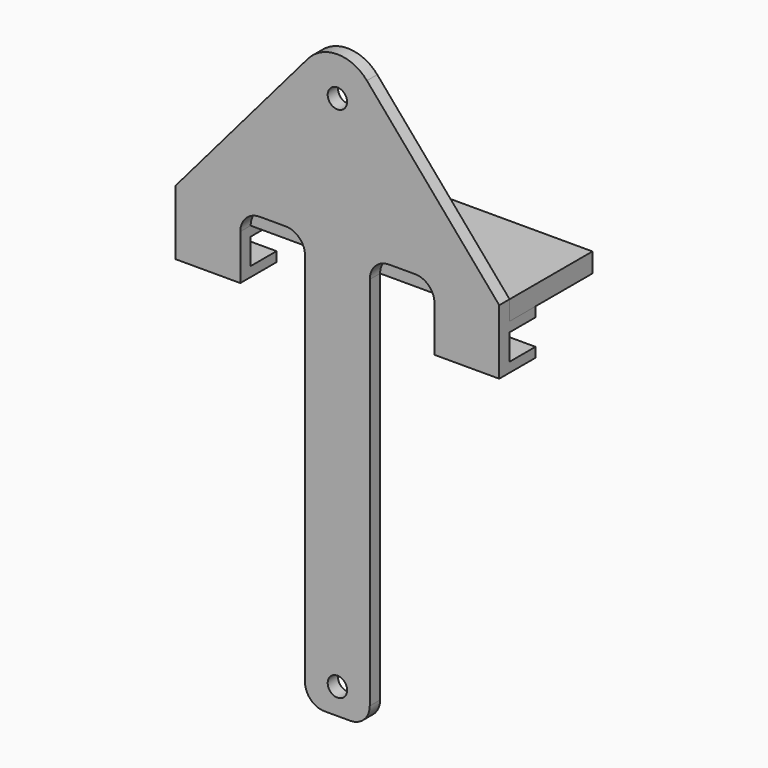
from build123d import *

# Parameters (mm, degrees)
F0_R     = 7.5
F1_DEPTH = 10
F2_W     = 50
F2_H     = 35
F3_DEPTH = 25
F5_DEPTH = 250.001
F6_W     = 250
F6_H     = 15
F7_DEPTH = 80


with BuildPart() as f1:
    # F0 (on Front) → F1 (new body)
    with BuildSketch(Plane.XZ):
        with BuildLine():
            Line((125, 50), (22.7990460802, 169.4988076003))
            ThreePointArc((22.7990460802, 169.4988076003), (0, 180), (-22.7990460802, 169.4988076003))
            Line((-22.7990460802, 169.4988076003), (-125, 50))
            Line((-125, 50), (-125, 0))
            Line((-125, 0), (-75, 0))
            Line((-75, 0), (-75, 35))
            ThreePointArc((-75, 35), (-70.6066017178, 45.6066017178), (-60, 50))
            Line((-60, 50), (-40, 50))
            ThreePointArc((-40, 50), (-29.3933982822, 45.6066017178), (-25, 35))
            Line((-25, 35), (-25, -255))
            ThreePointArc((-25, -255), (-20.6066017178, -265.6066017178), (-10, -270))
            Line((-10, -270), (0, -270))
            Line((0, -270), (10, -270))
            ThreePointArc((10, -270), (20.6066017178, -265.6066017178), (25, -255))
            Line((25, -255), (25, 35))
            ThreePointArc((25, 35), (29.3933982822, 45.6066017178), (40, 50))
            Line((40, 50), (60, 50))
            ThreePointArc((60, 50), (70.6066017178, 45.6066017178), (75, 35))
            Line((75, 35), (75, 0))
            Line((75, 0), (125, 0))
            Line((125, 0), (125, 50))
        make_face()
        with BuildLine():
            ThreePointArc((0, -242.5), (5.3033008589, -244.6966991411), (7.5, -250))
            ThreePointArc((7.5, -250), (-5.3033008589, -255.3033008589), (0, -242.5))
        make_face(mode=Mode.SUBTRACT)
        with Locations((0, 150)):
            Circle(F0_R, mode=Mode.SUBTRACT)
    extrude(amount=F1_DEPTH)

    # F2 (on face) → F3 (join)
    with BuildSketch(Plane(origin=(0, 0, 0), x_dir=(-1, 0, 0), z_dir=(0, 1, 0))):
        with Locations((-100, 17.5)):
            Rectangle(F2_W, F2_H)
        with Locations((100, 17.5)):
            Rectangle(F2_W, F2_H)
    extrude(amount=F3_DEPTH)

    # F4 (on face) → F5 (cut, through all)
    with BuildSketch(Plane.YZ.offset(125)):
        Polygon((25, 17.5), (25, 27.5), (0, 27.5), (0, 17.5), (0, 7.5), (25, 7.5), align=None)
    extrude(amount=-F5_DEPTH, mode=Mode.SUBTRACT)


with BuildPart() as f7:
    # F6 (on face) → F7 (new body)
    with BuildSketch(Plane(origin=(0, 0, 0), x_dir=(-1, 0, 0), z_dir=(0, 1, 0))):
        with Locations((0, 42.5)):
            Rectangle(F6_W, F6_H)
    extrude(amount=F7_DEPTH)


solid = Compound([f1.part, f7.part])
